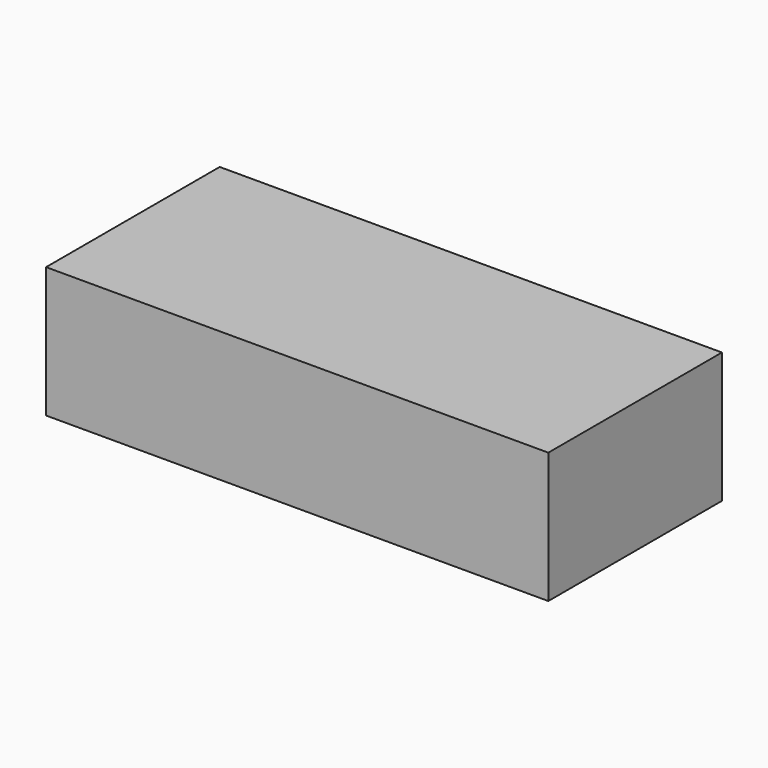
from build123d import *

# Parameters (mm, degrees)
F0_W     = 96.113152802
F0_H     = 41.5239520371
F1_DEPTH = 25


# Not quite as in the source:
# - the program builds the solid bodies; features that only make, move or delete a surface that nothing else refers to are left out


with BuildPart() as f1:
    # F0 (on Top) → F1 (new body)
    with BuildSketch(Plane.XY):
        Rectangle(F0_W, F0_H)
    extrude(amount=F1_DEPTH)


solid = f1.part
